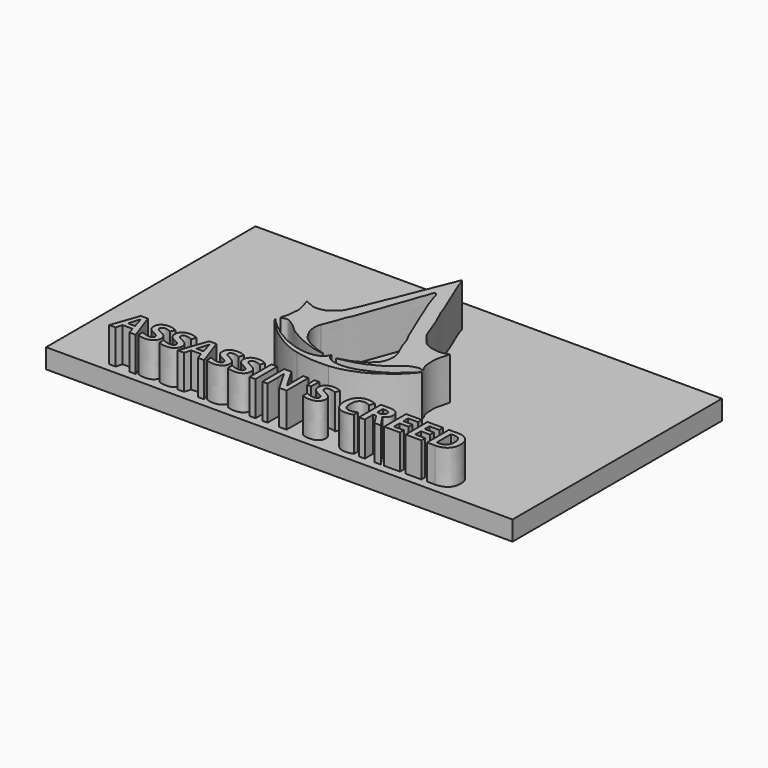
from build123d import *

# Parameters (mm, degrees)
F1_DEPTH     = 18
F2_DEPTH     = 18
F3_W         = 135.3224664927
F3_H         = 75.9391263127
F4_DEPTH     = 5.66829
F5_TEXT_SIZE = 11.0959478964
F6_DEPTH     = 10


# Not quite as in the source:
# - Text() gives the source's letters only with a copy of the font that has no kerning and outlines rounded to 1/6400 em; it was checked with that copy


with BuildPart() as f1:
    # F0 (on Top) → F1 (new body)
    with BuildSketch(Plane.XY):
        with BuildLine():
            add(Edge.make_bspline(
                [(-21.0363473743, -2.7983514592), (-20.3475792107, -3.1165628008), (-19.0678844055, -3.7077826368), (-17.5064024214, -4.1807127625), (-15.8276010067, -3.8657266795), (-14.5998683762, -3.6104863982), (-13.3389757009, -2.4211428115), (-12.1137192651, -1.6707785896), (-11.2538380862, 0.0198013782), (-10.7014648879, 1.1270886144), (-10.0430080427, 2.5972137746), (-9.5403835551, 4.1151315952), (-8.8015909888, 5.6492119815), (-8.0572057234, 7.5370724536), (-7.4917488773, 9.1693090036), (-6.6400964133, 10.7821672719), (-6.0957949818, 12.4992790991), (-5.5797449951, 13.691000625), (-5.3161596879, 14.2997018993)],
                knots=[0, 0, 0, 0, 0.0711972303, 0.1322806868, 0.1939112019, 0.2476850044, 0.3095836868, 0.3678968104, 0.4326380995, 0.4870637755, 0.5473941251, 0.6083849552, 0.6713439594, 0.7398215268, 0.8034041602, 0.8678695669, 0.93251111, 1, 1, 1, 1], degree=3))
            add(Edge.make_bspline(
                [(-11.3742006943, -9.7475349903), (-11.5197678174, -10.1281463078), (-11.8751680619, -11.057403906), (-11.5583769465, -13.9174240607), (-10.4737762264, -15.5789352453), (-9.7830219868, -16.7412160575), (-8.5651437101, -17.6878023894), (-7.6724747633, -18.3123029118), (-6.3937615147, -18.8206798121), (-5.2670026345, -19.4871471144), (-3.8994806634, -19.90599964), (-3.1016253154, -20.1231041866), (-1.8211195273, -20.534153687), (-2.8605318368, -20.4115359192), (-3.427214742, -20.2937017368), (-4.3982914814, -20.1296970445), (-5.4901928418, -19.9442661268), (-6.7066807448, -19.3459495964), (-8.2057800866, -19.0287133654), (-9.6572164178, -18.2471802908), (-11.3711336907, -17.5222957995), (-12.8759913221, -16.6154646985), (-13.9096079188, -16.0619376366), (-15.1030382381, -15.0622241009), (-16.068574896, -13.9921142304), (-17.3114071409, -13.2098251328), (-18.5073645596, -12.4111135808), (-19.5477354527, -12.3155255481), (-20.9319377261, -13.0844840838), (-20.5680553794, -11.8697552424), (-20.2395035695, -10.9561055128), (-20.0555833122, -9.7284610136), (-19.9460383682, -8.524439992), (-19.8395786528, -7.0905046765), (-20.1206810681, -6.0155566378), (-20.3523296896, -4.8335867016), (-20.8167763908, -3.686483385), (-20.9671073844, -3.0784169061), (-21.0363473743, -2.7983514592)],
                knots=[0, 0, 0, 0, 0.0286216775, 0.0698794547, 0.1046713741, 0.1331039567, 0.163153943, 0.1890839445, 0.2175555601, 0.2462136766, 0.2749983344, 0.2997400333, 0.3220067177, 0.3405452809, 0.3611048278, 0.3850136846, 0.4110377311, 0.4395676267, 0.4699276444, 0.5015035389, 0.5354287337, 0.5678577598, 0.5945763912, 0.6249364119, 0.6546550498, 0.6845995367, 0.7136568154, 0.7393779701, 0.7650549625, 0.7866837814, 0.8124925633, 0.8395006794, 0.8669535905, 0.8962343443, 0.9221643357, 0.9491919134, 0.9765986287, 1, 1, 1, 1], degree=3))
            add(Edge.make_bspline(
                [(20.5196812749, -2.8861910105), (20.3813581361, -3.4683200905), (20.1140004273, -4.5934875674), (19.6261756592, -6.0311236964), (19.421771687, -7.9677831559), (19.5889515295, -9.7687187515), (19.7232920512, -11.20758798), (20.9945938607, -13.2040930212), (19.4956451843, -12.3261181147), (18.5127150468, -12.6313975241), (17.4857780887, -12.8740320372), (16.07578323, -13.6220533077), (15.0613432192, -14.7317467731), (13.8149438842, -15.6646821835), (12.2107564056, -16.819236894), (10.4450980737, -17.7274808393), (8.5365641214, -18.663681454), (6.7629865556, -19.3146658623), (5.034695702, -19.7765766484), (3.2622031182, -20.1328960024), (1.0591825866, -20.6505843486), (2.2015588571, -20.2528194621), (2.9913638798, -20.0776487078), (3.7601596272, -19.7738013254), (4.550565503, -19.6164897928), (5.536644721, -19.2119759699), (6.8193197437, -18.5354539634), (7.5333590157, -18.0885207897), (8.7722535501, -17.3373787608), (9.561937661, -16.5788301459), (10.5673058496, -15.5941820484), (10.9958467766, -14.494789538), (11.4037181836, -13.3540417159), (11.453611372, -12.1470501916), (11.4561531585, -11.2485952062), (10.9620044127, -9.6372971463), (10.393045256, -8.4304663197), (9.689297468, -6.9954249939), (9.0926057517, -5.3328044198), (8.5762253012, -3.4202995324), (7.4636582323, -1.6498253137), (6.9730217357, -0.1103701709), (0.2644966974, 15.3437805033), (0.2823241019, 17.1807727942), (-1.0167854895, 19.3131135943), (-1.6109366641, 16.4798155994), (-2.6652055768, 14.4357112934), (-3.1438422513, 12.2361680596), (-3.9892063926, 10.3602033783), (-4.5806321011, 8.5521234813), (-5.3373834349, 6.435349402), (-6.0959985344, 4.2108039041), (-6.9493492244, 1.9060100139), (-7.7105711283, 0.0809929736), (-8.3990152056, -2.3293651551), (-9.1448250717, -3.374745189), (-9.6987669825, -5.5518604206), (-10.69578008, -7.9331031045), (-11.1605826246, -9.1762147373), (-11.3742006943, -9.7475349903)],
                knots=[0, 0, 0, 0, 0.0176211659, 0.0340590488, 0.0525846364, 0.0703294603, 0.087482209, 0.1039674005, 0.1170757925, 0.1309043061, 0.1445373468, 0.1611933487, 0.177535031, 0.194116331, 0.2127923413, 0.231705303, 0.2511389521, 0.2694515263, 0.2869794377, 0.3063965758, 0.3227058127, 0.3329591197, 0.345912707, 0.3578297533, 0.3696380731, 0.3835476289, 0.3994564812, 0.4119911792, 0.4276957738, 0.441965789, 0.4575117799, 0.4719656104, 0.4866604778, 0.5010605839, 0.5137854884, 0.5308129765, 0.5464757447, 0.5631273821, 0.5808866256, 0.5998837849, 0.6179202019, 0.6365495072, 0.6905042855, 0.7112531624, 0.7267603022, 0.7453986678, 0.7668871954, 0.7866453267, 0.8056474205, 0.8240062572, 0.8439100478, 0.8645430035, 0.885252629, 0.9044233791, 0.9251123205, 0.9401875917, 0.9598631091, 0.9815535322, 1, 1, 1, 1], degree=3))
            add(Edge.make_bspline(
                [(-5.3161596879, 14.2997018993), (-4.9693411513, 15.1868461257), (-4.3326303122, 16.8155201591), (-3.5433922401, 18.5497763733), (-2.7330414743, 20.696321074), (-1.8488511001, 22.9178684601), (-1.0985245397, 24.6523451347), (-0.659235341, 25.6894806953), (0.0660330394, 28.0295486681), (0.7598861745, 24.7818906914), (1.5092232258, 23.5475371577), (2.2776361682, 21.3022503483), (3.0821054969, 19.5579710975), (3.8287276824, 17.841077926), (4.7909603612, 15.106314482), (5.3042121209, 14.3410925534), (6.005121331, 11.8113084757), (7.3128779716, 9.1998935208), (8.1074848876, 7.5991074253), (8.9406022619, 5.0279793036), (9.6800938191, 3.3102854822), (10.3255545794, 1.2761697722), (11.4806235138, 0.0371901353), (12.6324402719, -1.7666680466), (14.4584779773, -2.9403249722), (16.4969766977, -3.4115760701), (18.5344629311, -3.5482496954), (19.8542650366, -3.1081034268), (20.5196812749, -2.8861910105)],
                knots=[0, 0, 0, 0, 0.0443720541, 0.0814609509, 0.1220704576, 0.1642991038, 0.2004708473, 0.231693191, 0.2632210378, 0.3028804255, 0.3388152055, 0.3792793566, 0.4165075812, 0.4544228059, 0.4993327051, 0.5256299812, 0.5683969503, 0.6148957967, 0.6513753792, 0.6949156248, 0.7326163912, 0.7710463298, 0.8060455439, 0.8450402877, 0.8843043644, 0.9230838583, 0.9612205122, 1, 1, 1, 1], degree=3))
        make_face()
    extrude(amount=F1_DEPTH)



with BuildPart() as f2:
    # F0 (on Top) → F2 (new body)
    with BuildSketch(Plane.XY):
        with BuildLine():
            add(Edge.make_bspline(
                [(-21.3053272714, -13.9416134006), (-21.1167703102, -14.1317275771), (-20.7174768193, -14.6372620684), (-20.0415233155, -15.2213802536), (-19.5136846792, -15.7659567676), (-18.7425948889, -16.3289003732), (-17.9146069918, -17.2072046653), (-17.0039994308, -17.6259669728), (-16.2629332825, -18.5125125196), (-15.1293006766, -18.9561326166), (-14.0871529896, -19.7178340575), (-12.9825545654, -20.3878258357), (-11.88336285, -20.8908582765), (-10.8348569393, -21.1125392637), (-9.6033120423, -21.7976354588), (-8.2817797002, -22.0096959315), (-6.3800406446, -22.5040355576), (-4.4471744241, -22.4940136551), (-2.8243335772, -22.2341647836), (-1.4355641437, -21.6295464574), (-0.6882201521, -20.8583185041), (-0.3992573299, -20.215076378), (-0.2546399483, -19.8931526393)],
                knots=[0.0381296916, 0.0381296916, 0.0381296916, 0.0381296916, 0.077207205, 0.1192865475, 0.1570410647, 0.1997203979, 0.2475941833, 0.2911455678, 0.3371835793, 0.3850913151, 0.4348170132, 0.4847386341, 0.5323727788, 0.5776168372, 0.6285838944, 0.6793455838, 0.7404684848, 0.8015013828, 0.8577335421, 0.910786493, 0.9553512673, 1, 1, 1, 1], degree=3))
            add(Edge.make_bspline(
                [(-17.5557099283, -18.07096228), (-17.9166941746, -17.7561728854), (-18.6034296664, -17.1562429661), (-19.3204529195, -16.3634903561), (-20.3815024671, -15.3211932892), (-20.9666844666, -14.8016189699), (-21.1358190971, -14.1578485174), (-21.3053272752, -13.941613404)],
                knots=[0, 0, 0, 0, 0.1924558227, 0.3652349836, 0.5629765016, 0.709252879, 0.8631316073, 0.8631316073, 0.8631316073, 0.8631316073], degree=3))
            add(Edge.make_bspline(
                [(-7.1932161227, -23.7036049366), (-7.6936961227, -23.6068576102), (-8.7089893497, -23.4105922145), (-10.208366746, -22.7093784509), (-11.7963089222, -22.0825028003), (-13.6841157061, -20.9683530529), (-14.9323627177, -19.9787093792), (-16.8415623768, -18.8084525785), (-17.3504747875, -18.2829057712), (-17.5557099283, -18.07096228)],
                knots=[0, 0, 0, 0, 0.1365275028, 0.2769650113, 0.4225298354, 0.5834198866, 0.7268677913, 0.8898507363, 1, 1, 1, 1], degree=3))
            add(Edge.make_bspline(
                [(2.6167279575, -24.5267856391), (2.1605711377, -24.5268881045), (1.3144645591, -24.5270781635), (0.3706558724, -24.5257998411), (-0.6625153675, -24.5304512882), (-1.4660013831, -24.5143249555), (-2.4140233212, -24.5775240468), (-3.3795104606, -24.3185641937), (-4.6507443594, -24.2447759061), (-6.0912783659, -23.9864923457), (-6.8425005426, -23.7936399873), (-7.1932161227, -23.7036049366)],
                knots=[0, 0, 0, 0, 0.1217971863, 0.2259166061, 0.3328891395, 0.4289870113, 0.5311600978, 0.6370108727, 0.7576069684, 0.886836391, 1, 1, 1, 1], degree=3))
            add(Edge.make_bspline(
                [(14.8235950619, -18.9170725644), (15.1082461259, -18.7357007423), (15.6535307731, -18.3882603758), (16.3322465674, -17.8999847436), (16.9638564614, -17.2491394008), (17.7932678095, -16.6490365236), (18.5180002724, -16.0044498259), (19.2858149435, -15.3525698019), (19.923198763, -14.6652568881), (20.6082967604, -14.0593901549), (21.2059213235, -13.373434189), (20.4693534201, -14.3752804889), (20.1398787648, -14.9002871673), (19.5310420648, -15.450059583), (18.9008490574, -16.1187626086), (18.3337967048, -16.7600505407), (17.5247294098, -17.578591674), (16.7116137712, -18.4314123143), (15.7779872995, -18.8869724856), (14.8072817916, -19.5920968391), (13.9788502682, -20.2747820793), (12.8787563043, -20.997131543), (11.6460507795, -21.7120693519), (10.1588739575, -22.4555775101), (8.6127649536, -23.1206757801), (7.1669545845, -23.5686782132), (5.9922870696, -23.9579587946), (4.2564951122, -24.3136063049), (3.1592834043, -24.4562502532), (2.6167279575, -24.5267856391)],
                knots=[0, 0, 0, 0, 0.0352092349, 0.0674476847, 0.1010322667, 0.1368413897, 0.1718950922, 0.2072716823, 0.2415624001, 0.2775980532, 0.3016573015, 0.3334610948, 0.3641598931, 0.3954629035, 0.4293984171, 0.4622462179, 0.5002663124, 0.5386151423, 0.5746434018, 0.6131219125, 0.649971746, 0.6902686037, 0.732700711, 0.7784345715, 0.8247228829, 0.8678785659, 0.9073282706, 0.9541751595, 1, 1, 1, 1], degree=3))
            add(Edge.make_bspline(
                [(-0.2546399483, -19.8931526393), (-0.1844983311, -20.1546503221), (-0.0455930942, -20.6725083225), (0.4401493889, -21.2841488419), (1.2003902161, -21.8832530333), (2.0963283942, -22.2375724493), (3.0258455655, -22.3482564776), (4.4350697657, -22.5445808513), (6.0807577709, -22.3556034221), (7.2949373683, -22.1767536686), (8.7959341024, -21.7684970622), (9.9326723844, -21.2646997507), (11.1362618248, -20.7046031278), (12.2730715189, -20.3340057315), (13.0060403054, -19.8993999512), (14.0562680704, -19.28464946), (14.5827758477, -19.0324335254), (14.8235950619, -18.9170725644)],
                knots=[0, 0, 0, 0, 0.0563503362, 0.1115936176, 0.1735650159, 0.2349255473, 0.2956465597, 0.3711517165, 0.4523725505, 0.5231900957, 0.6010887264, 0.6721961353, 0.7451534199, 0.8135536576, 0.8723752976, 0.9416257805, 1, 1, 1, 1], degree=3))
        make_face()
    extrude(amount=F2_DEPTH)


with BuildPart() as f1_1:
    add(f1.part)

    add(f2.part)  # F4 merges F2
    # F3 (on Top) → F4 (join)
    with BuildSketch(Plane.XY):
        with Locations((-0.2471506596, -0.8140206337)):
            Rectangle(F3_W, F3_H)
    extrude(amount=F4_DEPTH)

    # F5 (on face) → F6 (join)
    with BuildSketch(Plane.XY.offset(5.66829)):
        with Locations((-51.5253543854, -36.3668669015)):
            Text("ASSASSIN'S CREED", F5_TEXT_SIZE, font='Open Sans', font_style=FontStyle.BOLD, text_align=(TextAlign.LEFT, TextAlign.BOTTOM))
    extrude(amount=F6_DEPTH)


solid = f1_1.part
